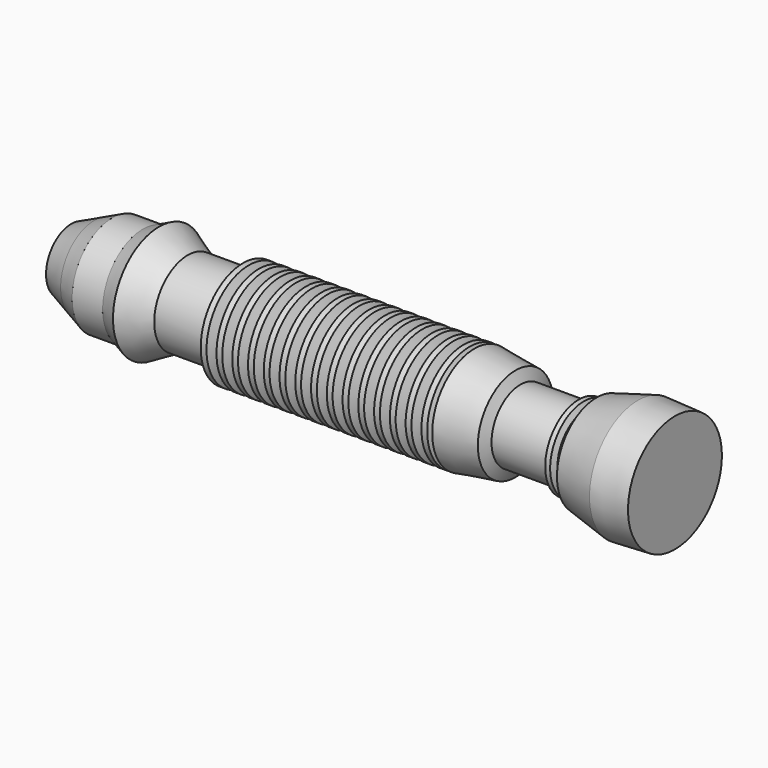
from build123d import *


# Not quite as in the source:
# - ends of sketch curves that miss each other by under 0.0002 mm in the source are joined


with BuildPart() as f1:
    # F0 (on Top) → F1 (revolve)
    with BuildSketch(Plane.XY):
        Polygon((146.7320563859, 15.8944390714), (152.7014625293, 15.8944390714), (150.8130326557, 20.0461714163), (149.7167594576, 20.0461714163), (148.6204862595, 20.0461714163), align=None)
        Polygon((0, 11.9488890163), (0, 0), (228.6, 0), (228.6, 22.225), (214.5352959633, 22.8744763881), (198.8992244005, 18.7337379903), (195.0535178185, 13.6998556554), (194.0553039312, 15.8944390714), (192.1773850918, 15.8944390714), (191.1042779684, 13.6998556554), (170.0893342495, 13.6998556554), (168.2125550841, 17.8259737997), (152.7014625293, 20.0461714163), (152.7014625293, 15.8944390714), (146.7320563859, 15.8944390714), (144.8436262557, 20.0461714163), (142.6510798595, 20.0461714163), (140.7626499859, 15.8944390714), (138.8742198557, 20.0461714163), (136.6816734595, 20.0461714163), (134.7932435859, 15.8944390714), (132.9048134557, 20.0461714163), (130.7122670595, 20.0461714163), (128.8238371859, 15.8944390714), (126.9354070557, 20.0461714163), (124.7428606595, 20.0461714163), (122.8544307859, 15.8944390714), (120.9660006557, 20.0461714163), (118.7734542595, 20.0461714163), (116.8850243859, 15.8944390714), (114.9965942557, 20.0461714163), (112.8040478595, 20.0461714163), (110.9156179859, 15.8944390714), (109.0271878557, 20.0461714163), (106.8346414595, 20.0461714163), (104.9462115859, 15.8944390714), (103.0577814557, 20.0461714163), (100.8652350595, 20.0461714163), (98.9768051859, 15.8944390714), (97.0883750557, 20.0461714163), (94.8958286595, 20.0461714163), (93.0073987859, 15.8944390714), (91.1189686557, 20.0461714163), (88.9264222595, 20.0461714163), (87.0379923859, 15.8944390714), (85.1495622557, 20.0461714163), (82.9570158595, 20.0461714163), (81.0685859859, 15.8944390714), (79.1801558557, 20.0461714163), (76.9876094595, 20.0461714163), (75.0991795859, 15.8944390714), (73.2107494557, 20.0461714163), (71.0182030595, 20.0461714163), (69.1297731859, 15.8944390714), (67.2413430557, 20.0461714163), (65.0487966595, 20.0461714163), (63.1603667859, 15.8944390714), (44.1223569214, 15.8944390714), (33.2462452351, 21.8172539027), (27.0914943445, 19.0177440883), (15.54095, 19.0177440883), (8.674332053, 15.8944390714), align=None)
    revolve(axis=Axis((114.3, 0, 0), (1, 0, 0)))


solid = f1.part
